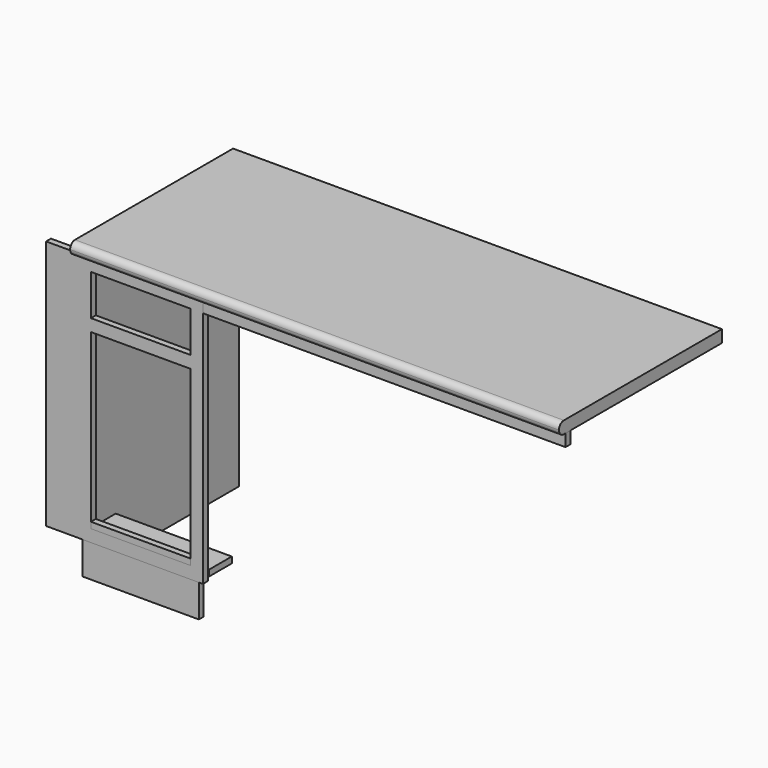
from build123d import *

# Parameters (mm, degrees)
F3_W      = 393.7
F3_H      = 781.05
F3_W_2    = 317.5
F3_H_2    = 520.7
F3_H_3    = 127
F4_DEPTH  = 19.05
F7_DEPTH  = 12.7
F8_W      = 361.95
F8_H      = 101.6
F9_DEPTH  = 19.05
F10_W     = 361.95
F10_H     = 88.9
F11_DEPTH = 19.05
F12_W     = 1130.3
F12_H     = 38.1
F13_DEPTH = 19.05
F14_W     = 1524
F14_H     = 635
F15_DEPTH = 38.1
F16_R     = 19.04999
F17_W     = 488.95
F17_H     = 781.05
F17_W_2   = 311.15
F17_H_2   = 539.75
F17_H_3   = 127
F18_DEPTH = 19.05


# Not quite as in the source:
# - a variable given as a bare number and used for a length is read in inches; the dataset says mm whatever the document's units were
# - a fillet or chamfer is up to 0.001 mm smaller than in the source, because OpenCascade refuses the exact size


with BuildPart() as f4:
    # F3 (on Front) → F4 (new body)
    with BuildSketch(Plane.XZ):
        with Locations((196.85, 390.525)):
            Rectangle(F3_W, F3_H)
        with Locations((196.85, 317.5)):
            Rectangle(F3_W_2, F3_H_2, mode=Mode.SUBTRACT)
        with Locations((196.85, 679.45)):
            Rectangle(F3_W_2, F3_H_3, mode=Mode.SUBTRACT)
    extrude(amount=F4_DEPTH)


with BuildPart() as f7:
    # F6 (on offset) → F7 (new body)
    with BuildSketch(Plane.YZ.offset(6.35)):
        Polygon((590.55, 781.05), (0, 781.05), (0, 0), (57.15, 0), (57.15, -101.6), (590.55, -101.6), align=None)
    extrude(amount=F7_DEPTH)


with BuildPart() as f9:
    # F8 (on Front) → F9 (new body)
    with BuildSketch(Plane.XZ):
        with Locations((200.025, -50.8)):
            Rectangle(F8_W, F8_H)
    extrude(amount=F9_DEPTH)


with BuildPart() as f11:
    # F10 (on Top) → F11 (new body)
    with BuildSketch(Plane.XY):
        with Locations((200.025, 64.8930611602)):
            Rectangle(F10_W, F10_H)
    extrude(amount=F11_DEPTH)


with BuildPart() as f13:
    # F12 (on face) → F13 (new body, through all)
    with BuildSketch(Plane.XZ.offset(19.05)):
        with Locations((958.85, 762)):
            Rectangle(F12_W, F12_H)
    extrude(amount=-F13_DEPTH)


with BuildPart() as f15:
    # F14 (on face) → F15 (new body)
    with BuildSketch(Plane.XY.offset(781.05)):
        with Locations((762, 273.05)):
            Rectangle(F14_W, F14_H)
    extrude(amount=F15_DEPTH)

    # F16 (radius 19.05 in the source; OpenCascade refuses exactly that, so slightly less here)
    f16_edges = [f15.edges().sort_by_distance(p)[0] for p in [
        (762, -44.45, 819.15),
        (762, -44.45, 781.05),
    ]]
    fillet(f16_edges, radius=F16_R)


with BuildPart() as f18:
    # F17 (on face) → F18 (new body)
    with BuildSketch(Plane.XZ):
        with Locations((149.225, 390.525)):
            Rectangle(F17_W, F17_H)
        with Locations((200.025, 307.975)):
            Rectangle(F17_W_2, F17_H_2, mode=Mode.SUBTRACT)
        with Locations((200.025, 679.45)):
            Rectangle(F17_W_2, F17_H_3, mode=Mode.SUBTRACT)
    extrude(amount=F18_DEPTH)


solid = Compound([f4.part, f7.part, f9.part, f11.part, f13.part, f15.part, f18.part])
